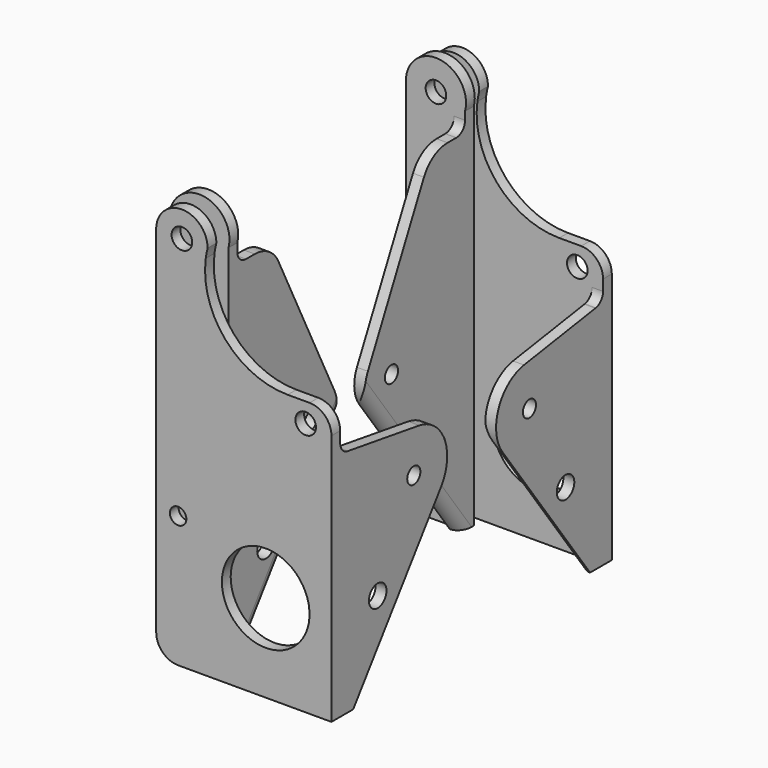
from build123d import *

# Parameters (mm, degrees)
F0_DEPTH       = 3.175
F20_DEPTH      = 3.175
F1_D           = 25.4
F21_D          = 6.35
F22_D          = 4.7625
F2_D           = 5.969
F3_D           = 5.969
F4_DEPTH       = 25.4
F8_DEPTH       = 3.175
F9_D           = 5.969
F12_DEPTH      = 3.175
F13_D          = 4.7752
F13_DEPTH      = 12.7
F13_TIP        = 1.434614814
F14_D          = 6.35
F14_DEPTH      = 12.7
F14_TIP        = 1.9077324654
F15_D          = 4.7752
F15_2_D        = 4.7752
F15_3_D        = 4.7752
F17_T1_DEPTH   = 70.262440232
F17_2_T1_DEPTH = 70.262440232
F17_3_T1_DEPTH = 71.7466703824
F17_4_T1_DEPTH = 71.7466703824


# Not quite as in the source:
# - a fillet or chamfer that OpenCascade refuses, or shapes differently, is made with other operations: its cross-section is extruded or revolved along the edge and cut away or added
# - a feature names something its author has since deleted; it is built from what else it names


with BuildPart() as f0:
    # F18 (on Front) → F0 (new body)
    with BuildSketch(Plane.XZ):
        with BuildLine():
            Line((-44.45, 0), (-19.05, 0))
            Line((-19.05, 0), (0, 0))
            Line((0, 0), (0, 73.025))
            ThreePointArc((0, 73.025), (-1.8598719395, 77.5151280605), (-6.35, 79.375))
            Line((-6.35, 79.375), (-12.7, 79.375))
            ThreePointArc((-12.7, 79.375), (-30.7094245393, 87.5400395149), (-36.4362123554, 106.4665062699))
            ThreePointArc((-36.4362123554, 106.4665062699), (-36.2084930614, 107.8649099863), (-35.8984617385, 109.2473967348))
            ThreePointArc((-35.8984617385, 109.2473967348), (-43.6106241383, 116.7024491997), (-50.8, 108.7420389807))
            Line((-50.8, 108.7420389807), (-50.8, 6.35))
            ThreePointArc((-50.8, 6.35), (-48.9401280605, 1.8598719395), (-44.45, 0))
        make_face()
    extrude(amount=-F0_DEPTH)

    # F19 (on Right) → F20 (join)
    with BuildSketch(Plane.YZ):
        with BuildLine():
            Line((0, 69.8649448027), (0, 0))
            Line((0, 0), (7.874, 0))
            Line((7.874, 0), (39.8421352783, 44.0003634282))
            ThreePointArc((39.8421352783, 44.0003634282), (40.960893879, 55.5554888764), (31.8310538657, 62.7261629214))
            Line((31.8310538657, 62.7261629214), (5.9537976693, 66.6998176699))
            ThreePointArc((5.9537976693, 66.6998176699), (5.8681024272, 66.7117839894), (5.7827650898, 66.7260810579))
            ThreePointArc((5.7827650898, 66.7260810579), (3.907842937, 67.8210855416), (3.175035173, 69.8649448027))
            Line((3.175035173, 69.8649448027), (0, 69.8649448027))
        make_face()
    extrude(amount=-F20_DEPTH)

    # F1 (through all)
    with Locations(Plane.XZ):
        with Locations((-19.05, 25.4)):
            Hole(F1_D / 2)

    # F21 (through all)
    with Locations(Plane.YZ):
        with Locations((16.764, 25.4)):
            Hole(F21_D / 2)

    # F22 (through all)
    with Locations(Plane.YZ):
        with Locations((29.844999956, 50.8)):
            Hole(F22_D / 2)

    # F2 (through all)
    with Locations(Plane.XZ):
        with Locations((-43.3578, 109.2473967348)):
            Hole(F2_D / 2)

    # F3 (through all)
    with Locations(Plane.XZ):
        with Locations((-7.4633745437, 73.7254909395)):
            Hole(F3_D / 2)

    # F18 (on Front) → F4 (cut)
    with BuildSketch(Plane.XZ):
        with BuildLine():
            ThreePointArc((-6.35, 79.375), (-1.8598719395, 77.5151280605), (0, 73.025))
            Line((0, 73.025), (0, 79.375))
            Line((0, 79.375), (-6.35, 79.375))
        make_face()
    extrude(amount=-F4_DEPTH, mode=Mode.SUBTRACT)


with BuildPart() as f23_1:
    # F23: instance of F0
    add(f0.part.mirror(Plane.XZ.offset(-50.8)))

    # F15#2 (through all)
    with Locations(Plane.XZ):
        with Locations((-44.45, 38.1)):
            Hole(F15_2_D / 2)

    # F17#2: fillet of radius 3.175 on 1 edges, made by hand

    # F17_2_s2 → F17_2_t1 (cut)
    with BuildSketch(Plane(origin=(0, 37.0470820327, -50.990933916), x_dir=(1, 0, 0), z_dir=(0, -0.5877852523, 0.8090169944))):
        with BuildLine():
            ThreePointArc((-3.175, 79.0009268148), (-2.2450640303, 76.7558627845), (0, 75.8259268148))
            Line((0, 75.8259268148), (-3.175, 75.8259268148))
            Line((-3.175, 75.8259268148), (-3.175, 79.0009268148))
        make_face()
    extrude(amount=F17_2_T1_DEPTH, mode=Mode.SUBTRACT)


with BuildPart() as f8:
    # F7 (on offset) → F8 (new body)
    with BuildSketch(Plane.XZ.offset(-6.35)):
        with BuildLine():
            Line((-52.07, 109.2473967348), (-52.07, 6.35))
            ThreePointArc((-52.07, 6.35), (-50.2101280605, 1.8598719395), (-45.72, 0))
            Line((-45.72, 0), (-34.925, 0))
            Line((-34.925, 0), (-34.925, 107.0587183665))
            ThreePointArc((-34.925, 107.0587183665), (-42.2545800129, 117.8894644561), (-52.07, 109.2473967348))
        make_face()
    extrude(amount=-F8_DEPTH)

    # F9 (through all)
    with Locations(Plane.XZ):
        with Locations((-43.3578, 109.2473967348)):
            Hole(F9_D / 2)

    # F11 (on offset) → F12 (join)
    with BuildSketch(Plane.YZ.offset(-34.925)):
        with BuildLine():
            ThreePointArc((24.4205172977, 96.2821081653), (20.9075401005, 100.1619750301), (15.875, 101.6))
            Line((15.875, 101.6), (12.7, 101.6))
            ThreePointArc((12.7, 101.6), (10.4549368419, 102.5299350976), (9.525, 104.7749975333))
            Line((9.525, 104.7749975333), (6.3898560263, 104.7749950975))
            Line((6.3898560263, 104.7749950975), (6.35, 104.7826025007))
            Line((6.35, 104.7826025007), (6.35, 0))
            Line((6.35, 0), (11.0606384104, 0))
            Line((11.0606384104, 0), (43.9011822821, 45.2011308435))
            ThreePointArc((43.9011822821, 45.2011308435), (45.6856367243, 49.9873526203), (44.7408448962, 55.0072694478))
            Line((44.7408448962, 55.0072694478), (24.4205172977, 96.2821081653))
        make_face()
    extrude(amount=-F12_DEPTH)

    # F13
    with Locations(Plane.YZ.offset(-34.925)):
        with Locations((36.195, 50.8)):
            Hole(F13_D / 2, depth=F13_DEPTH)
            with Locations((0, 0, -(F13_DEPTH + F13_TIP / 2))):  # 118° drill point
                Cone(0, F13_D / 2, F13_TIP, mode=Mode.SUBTRACT)

    # F14
    with Locations(Plane.YZ.offset(-34.925)):
        with Locations((19.939, 25.4)):
            Hole(F14_D / 2, depth=F14_DEPTH)
            with Locations((0, 0, -(F14_DEPTH + F14_TIP / 2))):  # 118° drill point
                Cone(0, F14_D / 2, F14_TIP, mode=Mode.SUBTRACT)

    # F15#3 (through all)
    with Locations(Plane.XZ):
        with Locations((-44.45, 38.1)):
            Hole(F15_3_D / 2)


with BuildPart() as f0_1:
    add(f0.part)

    # F15 (through all)
    with Locations(Plane.XZ):
        with Locations((-44.45, 38.1)):
            Hole(F15_D / 2)

    # F17: fillet of radius 3.175 on 1 edges, made by hand

    # F17_s2 → F17_t1 (cut)
    with BuildSketch(Plane(origin=(0, -1.9451453469, -2.6772628882), x_dir=(1, 0, 0), z_dir=(0, 0.5877852523, 0.8090169944))):
        with BuildLine():
            ThreePointArc((-3.175, 3.1951998137), (-2.2450640303, 5.440263844), (0, 6.3701998137))
            Line((0, 6.3701998137), (-3.175, 6.3701998137))
            Line((-3.175, 6.3701998137), (-3.175, 3.1951998137))
        make_face()
    extrude(amount=F17_T1_DEPTH, mode=Mode.SUBTRACT)


with BuildPart() as f16_1:
    # F16: instance of F8
    add(f8.part.mirror(Plane.XZ.offset(-50.8)))

    # F17#4: fillet of radius 3.175 on 1 edges, made by hand

    # F17_4_s2 → F17_4_t1 (cut)
    with BuildSketch(Plane(origin=(0, 35.9461255394, -49.4755973034), x_dir=(1, 0, 0), z_dir=(0, -0.5877852523, 0.8090169944))):
        with BuildLine():
            ThreePointArc((-34.925, 76.4228821859), (-35.8549359697, 74.1778181556), (-38.1, 73.2478821859))
            Line((-38.1, 73.2478821859), (-34.925, 73.2478821859))
            Line((-34.925, 73.2478821859), (-34.925, 76.4228821859))
        make_face()
    extrude(amount=F17_4_T1_DEPTH, mode=Mode.SUBTRACT)


with BuildPart() as f8_1:
    add(f8.part)

    # F17#3: fillet of radius 3.175 on 1 edges, made by hand

    # F17_3_s2 → F17_3_t1 (cut)
    with BuildSketch(Plane(origin=(0, -0.8441888536, -1.1619262756), x_dir=(1, 0, 0), z_dir=(0, 0.5877852523, 0.8090169944))):
        with BuildLine():
            ThreePointArc((-34.925, 5.7732444426), (-35.8549359697, 8.0183084729), (-38.1, 8.9482444426))
            Line((-38.1, 8.9482444426), (-34.925, 8.9482444426))
            Line((-34.925, 8.9482444426), (-34.925, 5.7732444426))
        make_face()
    extrude(amount=F17_3_T1_DEPTH, mode=Mode.SUBTRACT)


solid = Compound([f23_1.part, f0_1.part, f16_1.part, f8_1.part])
